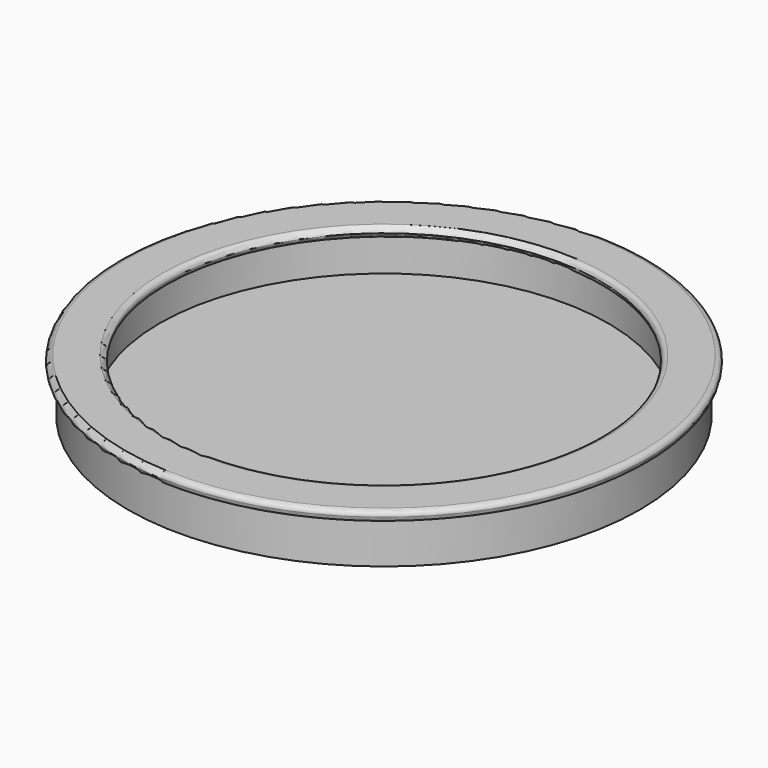
from build123d import *

# Parameters (mm, degrees)
F2_R = 2.53999


# Not quite as in the source:
# - a fillet or chamfer is up to 0.001 mm smaller than in the source, because OpenCascade refuses the exact size


with BuildPart() as f1:
    # F0 (on Front) → F1 (revolve)
    with BuildSketch(Plane.XZ):
        Polygon((-123.19, 0), (0, 0), (0, 3.81), (-107.95, 3.81), (-107.95, 20.32), (-104.14, 20.32), (-104.14, 25.4), (-127, 25.4), (-127, 20.32), (-123.19, 20.32), align=None)
    revolve(axis=Axis((0, 0, 1.905), (0, 0, -1)))

    # F2 (radius 2.54 in the source; OpenCascade refuses exactly that, so slightly less here)
    f2_edges = [f1.edges().sort_by_distance(p)[0] for p in [
        (127, 0, 25.4),
        (127, 0, 20.32),
        (-127, 0, 22.86),
        (104.14, 0, 20.32),
        (104.14, 0, 25.4),
        (-104.14, 0, 22.86),
    ]]
    fillet(f2_edges, radius=F2_R)


solid = f1.part
